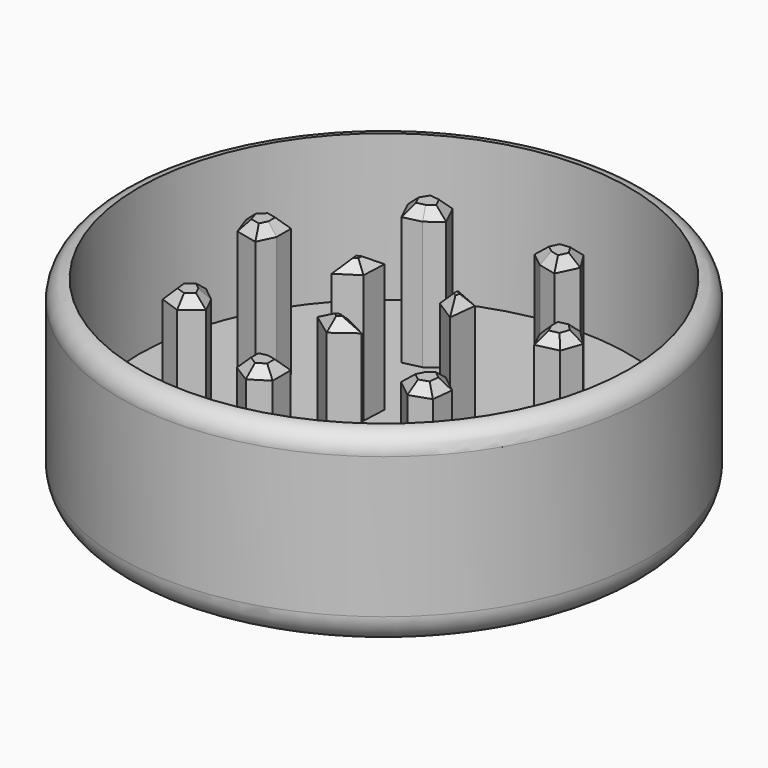
from build123d import *

# Parameters (mm, degrees)
F0_R      = 25
F1_DEPTH  = 4
F3_R      = 27
F4_DEPTH  = 4.4
F5_DEPTH  = 14.5
F6_R      = 27
F6_R_2    = 25.1
F7_DEPTH  = 15
F9_R      = 3
F10_SIZE  = 1
F11_R     = 3
F12_DEPTH = 3


# Not quite as in the source:
# - a fillet or chamfer that OpenCascade refuses, or shapes differently, is made with other operations: its cross-section is extruded or revolved along the edge and cut away or added
# - a feature names something its author has since deleted; it is built from what else it names


with BuildPart() as f1:
    # F0 (on Top) → F1 (new body)
    with BuildSketch(Plane.XY):
        Circle(F0_R)
    extrude(amount=F1_DEPTH)

    # F3 (on face) → F4 (join)
    with BuildSketch(Plane(origin=(0, 0, 0), x_dir=(1, 0, 0), z_dir=(0, 0, -1))):
        Circle(F3_R)
    extrude(amount=-F4_DEPTH)

    # F2 (on face) → F5 (join)
    with BuildSketch(Plane.XY.offset(4)):
        Polygon((1.8290777225, -14.20661062), (0, -13.8), (-1.8290777225, -14.20661062), (-1.8290777225, -16.5130756795), (0, -17.6663082093), (1.8290777225, -16.5130756795), align=None)
        Polygon((10.7892744581, -8.6041592657), (9.9667641351, -10.2877073879), (11.7700311319, -11.7257648309), (13.812075937, -11.014763005), (14.0508537454, -8.8657037362), (12.2475867487, -7.4276462932), align=None)
        Polygon((13.4540051881, 3.0707888886), (14.257429314, 1.3780493383), (16.506066479, 1.8912860975), (17.2233769785, 3.9311234023), (15.6920503129, 5.4577239479), (13.4434131479, 4.9444871887), align=None)
        Polygon((5.9875955998, 12.4333703771), (7.811959421, 12.0061068057), (8.8126971051, 14.0841600192), (7.6651238623, 15.9167937073), (5.5168129352, 15.671374182), (4.5160752511, 13.5933209684), align=None)
        Polygon((-5.9875955998, 12.4333703771), (-4.5160752511, 13.5933209684), (-5.5168129352, 15.671374182), (-7.6651238623, 15.9167937073), (-8.8126971051, 14.0841600192), (-7.811959421, 12.0061068057), align=None)
        Polygon((-13.4540051881, 3.0707888886), (-13.4434131479, 4.9444871887), (-15.6920503129, 5.4577239479), (-17.2233769785, 3.9311234023), (-16.506066479, 1.8912860975), (-14.257429314, 1.3780493383), align=None)
        Polygon((-10.7892744581, -8.6041592657), (-12.2475867487, -7.4276462932), (-14.0508537454, -8.8657037362), (-13.812075937, -11.014763005), (-11.7700311319, -11.7257648309), (-9.9667641351, -10.2877073879), align=None)
        Polygon((2.2625249746, -5.6745974369), (0, -4.5038154349), (-2.2625249746, -5.6745974369), (0, -7.3385047726), align=None)
        Polygon((3.7830830493, 4.7967028232), (3.9004185806, 2.2519077174), (6.0456080239, 0.8778946137), (6.3553315589, 3.6692523863), align=None)
        Polygon((-6.0456080239, 0.8778946137), (-3.9004185806, 2.2519077174), (-3.7830830493, 4.7967028232), (-6.3553315589, 3.6692523863), align=None)
    extrude(amount=F5_DEPTH)

    # F6 (on face) → F7 (join)
    with BuildSketch(Plane.XY.offset(4.4)):
        Circle(F6_R)
        Circle(F6_R_2, mode=Mode.SUBTRACT)
    extrude(amount=F7_DEPTH)

    # F8: fillet of radius 2 on 1 edges, made by hand

    # F8_s1 → F8_t2 (revolve, cut)
    with BuildSketch(Plane.XZ):
        with BuildLine():
            ThreePointArc((27, 17.4025015645), (26.4491376746, 18.7809064397), (25.1, 19.4))
            Line((25.1, 19.4), (27, 19.4))
            Line((27, 19.4), (27, 17.4025015645))
        make_face()
    revolve(axis=Axis((0, 0, 19.4), (0, 0, 1)), mode=Mode.SUBTRACT)

    # F9
    f9_edges = [f1.edges().sort_by_distance(p)[0] for p in [
        (-27, 0, 0),
    ]]
    fillet(f9_edges, radius=F9_R)

    # F10
    f10_edges = [f1.edges().sort_by_distance(p)[0] for p in [
        (1.131262, -5.089206, 18.5),
        (-1.131262, -5.089206, 18.5),
        (-1.131262, -6.506551, 18.5),
        (1.131262, -6.506551, 18.5),
        (6.20047, 2.273574, 18.5),
        (5.069207, 4.232978, 18.5),
        (3.841751, 3.524305, 18.5),
        (4.973013, 1.564901, 18.5),
        (5.016444, 14.632348, 18.5),
        (5.251835, 13.013346, 18.5),
        (6.899778, 12.219739, 18.5),
        (8.312328, 13.045133, 18.5),
        (8.23891, 15.000477, 18.5),
        (6.590968, 15.794084, 18.5),
        (-5.069207, 4.232978, 18.5),
        (-6.20047, 2.273574, 18.5),
        (-4.973013, 1.564901, 18.5),
        (-3.841751, 3.524305, 18.5),
        (-5.251835, 13.013346, 18.5),
        (-5.016444, 14.632348, 18.5),
        (-6.590968, 15.794084, 18.5),
        (-8.23891, 15.000477, 18.5),
        (-8.312328, 13.045133, 18.5),
        (-6.899778, 12.219739, 18.5),
        (13.855717, 2.224419, 18.5),
        (15.381748, 1.634668, 18.5),
        (16.864722, 2.911205, 18.5),
        (16.457714, 4.694424, 18.5),
        (14.567732, 5.201106, 18.5),
        (13.448709, 4.007638, 18.5),
        (10.378019, -9.445933, 18.5),
        (10.868398, -11.006736, 18.5),
        (12.791054, -11.370264, 18.5),
        (13.931465, -9.940233, 18.5),
        (13.14922, -8.146675, 18.5),
        (11.518431, -8.015903, 18.5),
        (0.914539, -14.003305, 18.5),
        (-0.914539, -14.003305, 18.5),
        (-1.829078, -15.359843, 18.5),
        (-0.914539, -17.089692, 18.5),
        (0.914539, -17.089692, 18.5),
        (1.829078, -15.359843, 18.5),
        (-11.518431, -8.015903, 18.5),
        (-13.14922, -8.146675, 18.5),
        (-13.931465, -9.940233, 18.5),
        (-12.791054, -11.370264, 18.5),
        (-10.868398, -11.006736, 18.5),
        (-10.378019, -9.445933, 18.5),
        (-15.381748, 1.634668, 18.5),
        (-13.855717, 2.224419, 18.5),
        (-13.448709, 4.007638, 18.5),
        (-14.567732, 5.201106, 18.5),
        (-16.457714, 4.694424, 18.5),
        (-16.864722, 2.911205, 18.5),
    ]]
    chamfer(f10_edges, length=F10_SIZE)

    # F11 (on face) → F12 (cut)
    with BuildSketch(Plane.XY.offset(4.4)):
        Circle(F11_R)
    extrude(amount=-F12_DEPTH, mode=Mode.SUBTRACT)


solid = f1.part
